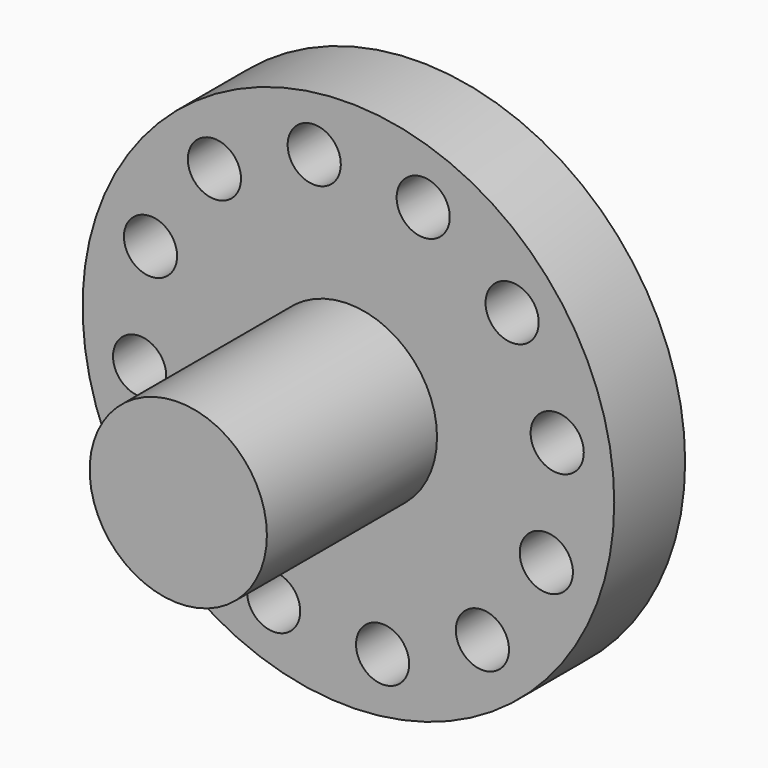
from build123d import *

# Parameters (mm, degrees)
F0_R            = 15
F2_DEPTH        = 5
F1_R            = 1.5
F3_DEPTH        = 6
F3_COPIES_COUNT = 12
F4_R            = 5
F5_DEPTH        = 17


# Not quite as in the source:
# - a pattern or mirror of a feature is missing from the dataset's text; its kind, count and spacing are read off the source's solid


with BuildPart() as f2:
    # F0 (on Front) → F2 (new body)
    with BuildSketch(Plane.XZ):
        Circle(F0_R)
    extrude(amount=F2_DEPTH)

    # F1 (on face) → F3 (cut)
    with BuildSketch(Plane.XZ):
        with Locations((-7.5604245067, 9.2375520617)):
            Circle(F1_R)
    f3 = extrude(amount=F3_DEPTH, mode=Mode.SUBTRACT)

    # F3_copies: F3 ×12 about axis
    f3_copies_axis = Axis((0, 0, 0), (0, 1, 0))
    for i in range(1, F3_COPIES_COUNT):
        add(f3.rotate(f3_copies_axis, i * 360 / F3_COPIES_COUNT), mode=Mode.SUBTRACT)

    # F4 (on face) → F5 (join)
    with BuildSketch(Plane.XZ):
        Circle(F4_R)
    extrude(amount=F5_DEPTH)


solid = f2.part
